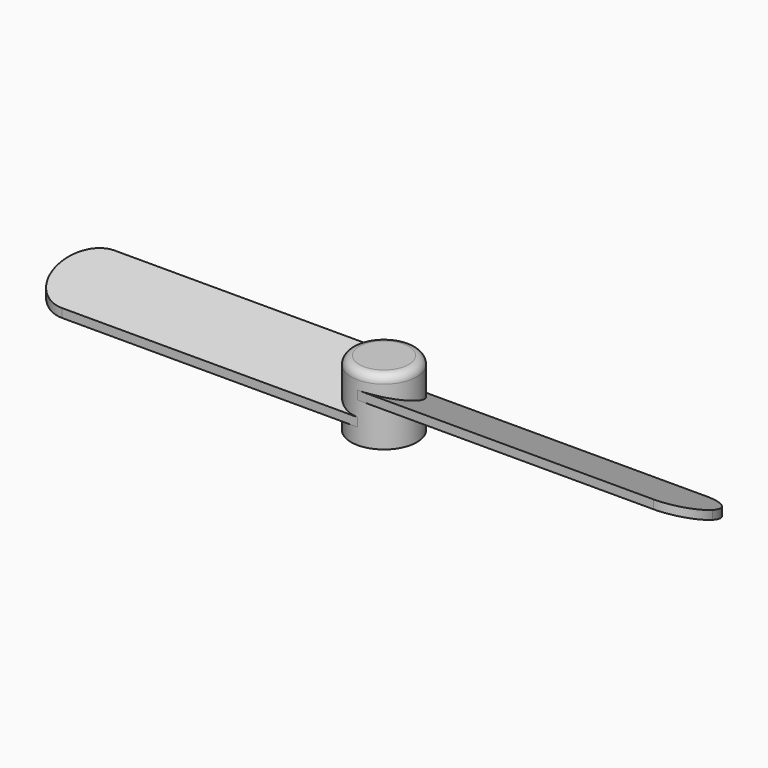
from build123d import *

# Parameters (mm, degrees)
F0_R        = 2
F1_DEPTH    = 4
F3_DEPTH    = 20
F5_DEPTH    = 20
F6_T1_DEPTH = 10.5320888862
F6_T3_DEPTH = 10.5320888862
F7_R        = 0.5
F8_R        = 0.25
F9_DEPTH    = 3


# Not quite as in the source:
# - a fillet or chamfer that OpenCascade refuses, or shapes differently, is made with other operations: its cross-section is extruded or revolved along the edge and cut away or added


with BuildPart() as f1:
    # F0 (on Top) → F1 (new body)
    with BuildSketch(Plane.XY):
        Circle(F0_R)
    extrude(amount=F1_DEPTH)

    # F2 (on Right) → F3 (join)
    with BuildSketch(Plane.YZ):
        Polygon((2, 1.5), (-2, 2.9558809371), (-2, 2.4237920508), (2, 0.9679111138), align=None)
    extrude(amount=F3_DEPTH)

    # F4 (on Right) → F5 (join)
    with BuildSketch(Plane.YZ):
        Polygon((2, 2.4237920508), (2, 2.9558809371), (-2, 1.5), (-2, 0.9679111138), align=None)
    extrude(amount=-F5_DEPTH)

    # F6: fillet of radius 2 on 4 edges, made by hand

    # F6_s2 → F6_t1 (cut)
    with BuildSketch(Plane.XY.offset(-2.5762079492)):
        with BuildLine():
            ThreePointArc((-18, 2), (-19.4142135624, 1.4142135624), (-20, 0))
            Line((-20, 0), (-20, 2))
            Line((-20, 2), (-18, 2))
        make_face()
        with BuildLine():
            ThreePointArc((18, -2), (19.4142135624, -1.4142135624), (20, 0))
            Line((20, 0), (20, -2))
            Line((20, -2), (18, -2))
        make_face()
    extrude(amount=F6_T1_DEPTH, mode=Mode.SUBTRACT)

    # F6_s4 → F6_t3 (cut)
    with BuildSketch(Plane.XY.offset(-4.0320888862)):
        with BuildLine():
            ThreePointArc((-18, -2), (-19.4142135624, -1.4142135624), (-20, 0))
            Line((-20, 0), (-20, -2))
            Line((-20, -2), (-18, -2))
        make_face()
        with BuildLine():
            ThreePointArc((18, 2), (19.4142135624, 1.4142135624), (20, 0))
            Line((20, 0), (20, 2))
            Line((20, 2), (18, 2))
        make_face()
    extrude(amount=F6_T3_DEPTH, mode=Mode.SUBTRACT)

    # F7
    f7_edges = [f1.edges().sort_by_distance(p)[0] for p in [
        (-2, 0, 4),
    ]]
    fillet(f7_edges, radius=F7_R)

    # F8 (on face) → F9 (cut)
    with BuildSketch(Plane(origin=(0, 0, 0), x_dir=(1, 0, 0), z_dir=(0, 0, -1))):
        Circle(F8_R)
    extrude(amount=-F9_DEPTH, mode=Mode.SUBTRACT)


solid = f1.part
